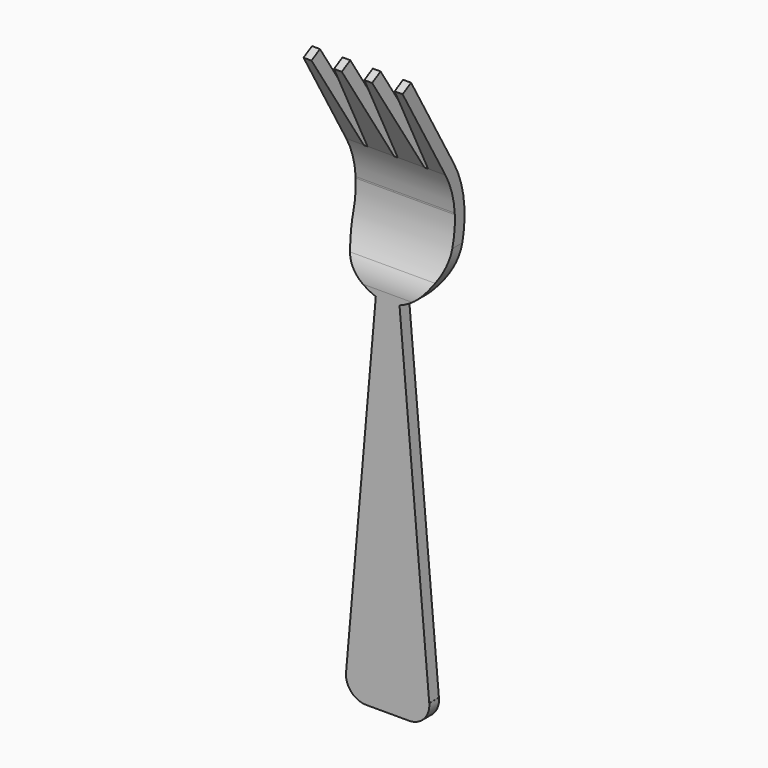
from build123d import *

# Parameters (mm, degrees)
F1_DEPTH     = 4.318
F1_FACE_W    = 8.4660017827
F1_FACE_H    = 4.318
F4_W         = 8.4660017827
F4_H         = 4.318
F5_DEPTH     = 0.508
F7_DEPTH     = 13.462
F9_T1_DEPTH  = 101.8009504956
F10_T1_DEPTH = 101.8156278686
F8_FACE_W    = 35.3900017827
F8_FACE_H    = 4.318
F14_DEPTH    = 45.466


# Not quite as in the source:
# - a fillet or chamfer that OpenCascade refuses, or shapes differently, is made with other operations: its cross-section is extruded or revolved along the edge and cut away or added


with BuildPart() as f1:
    # F0 (on Front) → F1 (new body)
    with BuildSketch(Plane.XZ):
        with BuildLine():
            ThreePointArc((-14.8547158409, -68.6793103814), (-12.973951869, -74.217922925), (-7.62, -76.5734910965))
            Line((-7.62, -76.5734910965), (7.62, -76.5734910965))
            ThreePointArc((7.62, -76.5734910965), (12.9819628095, -74.2196084737), (14.8784083325, -68.6793103814))
            Line((14.8784083325, -68.6793103814), (14.8547158409, -68.6793103814))
            Line((14.8547158409, -68.6793103814), (-14.8547158409, -68.6793103814))
        make_face()
        Polygon((-7.1831139455, 19.1512540919), (-14.8547158409, -68.6793103814), (14.8547158409, -68.6793103814), (7.1831139455, 19.1512540919), (4.2330008913, 52.9264810056), (-4.2330008913, 52.9264810056), align=None)
    extrude(amount=F1_DEPTH)

    # F3: sweep along a path in F2
    with BuildLine(Plane.YZ) as f3_path:
        Line((-4.318, 52.9264810056), (-4.318, 55.3578620488))
        ThreePointArc((-4.318, 55.3578620488), (-3.7519884271, 59.1070386053), (-2.1044055351, 62.5220297571))
        ThreePointArc((-2.1044055351, 62.5220297571), (2.3667917296, 72.1058812805), (3.5367051605, 82.6165005565))
    # F1_face (on face) → F3 (sweep)
    with BuildSketch(Plane(origin=(0, -2.159, 52.9264810056), x_dir=(1, 0, 0), z_dir=(0, 0, 1))):
        Rectangle(F1_FACE_W, F1_FACE_H)
    sweep(path=f3_path.line)

    # F4 (on face) → F5 (join)
    with BuildSketch(Plane(origin=(0, -4.2773000259, 82.2099457989), x_dir=(1, 0, 0), z_dir=(0, -0.0519587059, 0.9986492342))):
        with Locations((0, 9.9835743541)):
            Rectangle(F4_W, F4_H)
    extrude(amount=F5_DEPTH)

    # F6 (on face) → F7 (join)
    with BuildSketch(Plane.YZ.offset(4.2330008913)):
        with BuildLine():
            Line((-4.318, 52.9264810056), (0, 52.9264810056))
            Line((0, 52.9264810056), (0, 55.3578620488))
            ThreePointArc((0, 55.3578620488), (0.3735676381, 57.8323185761), (1.4609723468, 60.0862127363))
            ThreePointArc((1.4609723468, 60.0862127363), (6.5240819847, 70.938807275), (7.8488725536, 82.8408582485))
            Line((7.8488725536, 82.8408582485), (7.822477531, 83.3481720595))
            Line((7.822477531, 83.3481720595), (3.5103101379, 83.1238143674))
            Line((3.5103101379, 83.1238143674), (3.5367051605, 82.6165005565))
            ThreePointArc((3.5367051605, 82.6165005565), (2.3667917296, 72.1058812805), (-2.1044055351, 62.5220297571))
            ThreePointArc((-2.1044055351, 62.5220297571), (-3.7519884271, 59.1070386053), (-4.318, 55.3578620488))
            Line((-4.318, 55.3578620488), (-4.318, 52.9264810056))
        make_face()
    extrude(amount=F7_DEPTH)

    # F8: F1 across plane


with BuildPart() as f1_1:
    add(f1.part)
    add(f1.part.mirror(Plane.YZ))

    # F9: fillet of radius 20.8491483247 on 1 edges, made by hand

    # F9_s2 → F9_t1 (cut)
    with BuildSketch(Plane.XZ.offset(-48.7414752478)):
        with BuildLine():
            ThreePointArc((17.6950008913, 72.4230711047), (14.0025238199, 60.5767376056), (4.2330008913, 52.9264810056))
            Line((4.2330008913, 52.9264810056), (17.6950008913, 52.9264810056))
            Line((17.6950008913, 52.9264810056), (17.6950008913, 72.4230711047))
        make_face()
    extrude(amount=F9_T1_DEPTH, mode=Mode.SUBTRACT)

    # F10: fillet of radius 20.8534 on 1 edges, made by hand

    # F10_s2 → F10_t1 (cut)
    with BuildSketch(Plane.XZ.offset(-48.7488139343)):
        with BuildLine():
            ThreePointArc((-4.2330008913, 52.9264810056), (-14.0026048293, 60.5784652564), (-17.6950008913, 72.4260065793))
            Line((-17.6950008913, 72.4260065793), (-17.6950008913, 52.9264810056))
            Line((-17.6950008913, 52.9264810056), (-4.2330008913, 52.9264810056))
        make_face()
    extrude(amount=F10_T1_DEPTH, mode=Mode.SUBTRACT)

    # F12: sweep along a path in F11
    with BuildLine(Plane.YZ) as f12_path:
        ThreePointArc((5.6663938345, 83.2359932134), (4.2906494395, 90.7738508992), (1.2476332355, 97.8060641719))
        Line((1.2476332355, 97.8060641719), (-17.8702931298, 131.016411811))
    # F8_face (on face) → F12 (sweep)
    with BuildSketch(Plane(origin=(0, 5.6663938345, 83.2359932134), x_dir=(1, 0, 0), z_dir=(0, -0.0519587059, 0.9986492342))):
        Rectangle(F8_FACE_W, F8_FACE_H)
    sweep(path=f12_path.line)

    # F13 (on face) → F14 (cut)
    with BuildSketch(Plane(origin=(0, 41.3553334691, 23.8066830455), x_dir=(1, 0, 0), z_dir=(0, -0.8666583712, -0.4989020622))):
        Polygon((-6.7998209327, 122.4935306315), (-14.8516167313, 122.4935306315), (-11.232118832, 81.1224803329), (-10.419318832, 81.1224803329), align=None)
        Polygon((4.0258978993, 122.4935306315), (-4.0258978993, 122.4935306315), (-0.4064, 81.1224803329), (0, 81.1224803329), (0.4064, 81.1224803329), align=None)
        Polygon((11.232118832, 81.1224803329), (14.8516167313, 122.4935306315), (6.7998209327, 122.4935306315), (10.419318832, 81.1224803329), align=None)
    extrude(amount=-F14_DEPTH, mode=Mode.SUBTRACT)


solid = f1_1.part
